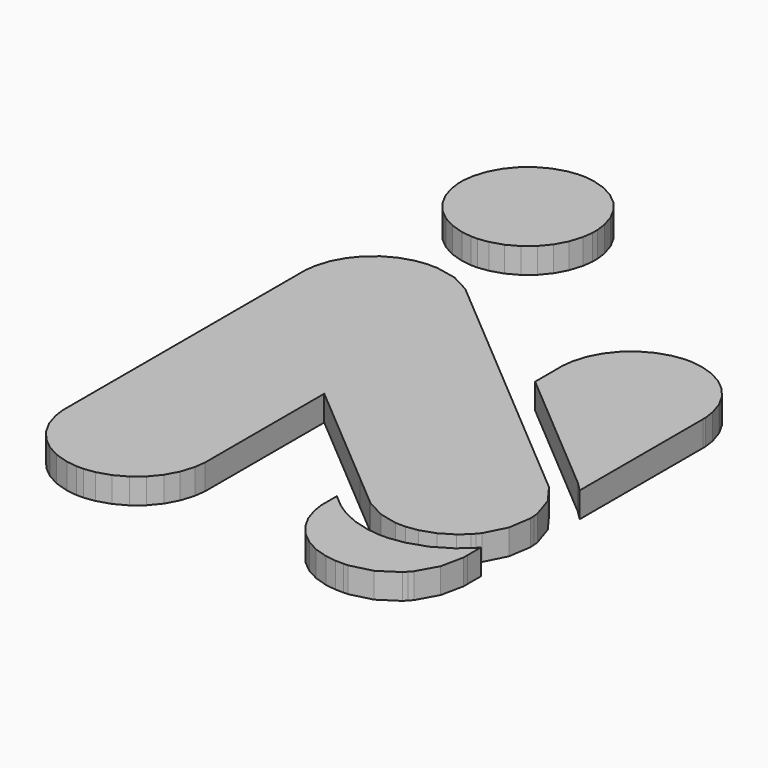
from build123d import *

# Parameters (mm, degrees)
F1_DEPTH = 0.15
F2_SCALE = 4


# Not quite as in the source:
# - ends of sketch curves that miss each other by under 0.0002 mm in the source are joined


with BuildPart() as f1:
    # F0 (on Top) → F1 (new body)
    with BuildSketch(Plane.XY):
        Polygon((-0.66371, 2.45638), (-0.68363, 2.45638), (-0.70359, 2.45638), (-0.76332, 2.44835), (-0.8376, 2.42524), (-0.90488, 2.38867), (-0.96346, 2.34027), (-1.01186, 2.28169), (-1.04843, 2.21441), (-1.07154, 2.14013), (-1.07957, 2.0804), (-1.07957, 2.06044), (-1.07957, 2.04052), (-1.07154, 1.9808), (-1.04843, 1.90652), (-1.01186, 1.8393), (-0.96346, 1.78065), (-0.90488, 1.73231), (-0.8376, 1.69574), (-0.76332, 1.67263), (-0.70359, 1.66455), (-0.68363, 1.66455), (-0.66371, 1.66455), (-0.60399, 1.67263), (-0.52971, 1.69574), (-0.46243, 1.73231), (-0.40384, 1.78065), (-0.35545, 1.8393), (-0.31893, 1.90652), (-0.29582, 1.9808), (-0.28774, 2.04052), (-0.28774, 2.06044), (-0.28774, 2.0804), (-0.29582, 2.14013), (-0.31893, 2.21441), (-0.35545, 2.28169), (-0.40384, 2.34027), (-0.46243, 2.38867), (-0.52971, 2.42524), (-0.60399, 2.44835), align=None)
    extrude(amount=F1_DEPTH)


with BuildPart() as f1b:
    # F0 (on Top) → F1, piece 2 (new body)
    with BuildSketch(Plane.XY):
        Polygon((-0.25009, -0.8451), (-0.25009, 0.01508), (0.41001, -0.54476), (0.57864, -0.68777), (0.59751, -0.70383), (0.70537, -0.76162), (0.81361, -0.78733), (0.84973, -0.78733), (0.87241, -0.78733), (0.94057, -0.7774), (1.02601, -0.74859), (1.10332, -0.70215), (1.15491, -0.65663), (1.16962, -0.63938), (1.18773, -0.61801), (1.24932, -0.49653), (1.2701, -0.36192), (1.26782, -0.33404), (1.26548, -0.3061), (1.22305, -0.17665), (1.14254, -0.06679), (1.12122, -0.04872), (0.31979, 0.63091), (-0.37688, 1.22178), (-0.39603, 1.23801), (-0.50518, 1.29606), (-0.62671, 1.32117), (-0.652, 1.32091), (-0.65352, 1.32085), (-0.65764, 1.32102), (-0.65861, 1.32108), (-0.66649, 1.32128), (-0.6694, 1.32128), (-0.69052, 1.32128), (-0.75384, 1.31277), (-0.8325, 1.28835), (-0.90368, 1.24967), (-0.96574, 1.19845), (-1.01702, 1.1364), (-1.0557, 1.06522), (-1.08017, 0.9866), (-1.08868, 0.92334), (-1.08868, 0.90223), (-1.08868, -0.8451), (-1.08868, -0.86616), (-1.08017, -0.92948), (-1.0557, -1.00809), (-1.01702, -1.07927), (-0.96574, -1.14133), (-0.90368, -1.19255), (-0.8325, -1.23123), (-0.75384, -1.25565), (-0.69052, -1.26422), (-0.6694, -1.26422), (-0.64836, -1.26422), (-0.58504, -1.25565), (-0.50638, -1.23123), (-0.43514, -1.19255), (-0.37309, -1.14133), (-0.32181, -1.07927), (-0.28313, -1.00809), (-0.25866, -0.92948), (-0.25009, -0.86616), align=None)
    extrude(amount=F1_DEPTH)


with BuildPart() as f1c:
    # F0 (on Top) → F1, piece 3 (new body)
    with BuildSketch(Plane.XY):
        Polygon((0.85348, 1.32128), (0.84996, 1.32128), (0.8288, 1.32112), (0.76543, 1.31201), (0.68687, 1.28678), (0.61596, 1.2474), (0.55428, 1.19558), (0.50361, 1.13302), (0.46557, 1.06147), (0.4418, 0.98258), (0.43389, 0.91916), (0.43411, 0.89806), (0.43416, 0.71609), (1.21107, 0.05719), (1.21665, 0.05246), (1.26819, 0.00135), (1.27291, -0.00413), (1.27265, 0.90658), (1.27243, 0.92746), (1.26337, 0.99002), (1.23847, 1.06776), (1.19946, 1.13819), (1.14814, 1.19959), (1.08618, 1.25033), (1.01526, 1.28863), (0.93714, 1.31288), (0.87437, 1.32128), align=None)
    extrude(amount=F1_DEPTH)


with BuildPart() as f1d:
    # F0 (on Top) → F1, piece 4 (new body)
    with BuildSketch(Plane.XY):
        Polygon((1.14407, -1.15072), (1.16229, -1.13102), (1.18041, -1.11133), (1.2453, -0.99469), (1.2734, -0.86035), (1.27314, -0.83181), (1.27308, -0.73199), (1.25355, -0.75467), (1.18508, -0.8144), (1.08276, -0.87538), (0.96975, -0.9132), (0.87975, -0.92622), (0.84973, -0.92622), (0.82522, -0.92622), (0.75182, -0.91748), (0.65753, -0.89198), (0.56908, -0.85048), (0.50746, -0.80952), (0.48879, -0.79373), (0.43454, -0.74773), (0.43459, -0.84034), (0.43476, -0.86117), (0.44382, -0.92367), (0.46878, -1.00147), (0.50778, -1.07188), (0.55911, -1.1333), (0.62107, -1.18403), (0.69197, -1.22233), (0.7701, -1.24659), (0.83282, -1.25505), (0.85376, -1.25505), (0.85673, -1.25505), (0.8658, -1.25505), (0.87562, -1.25505), (0.87893, -1.25505), (0.90643, -1.25477), (1.03458, -1.22223), align=None)
    extrude(amount=F1_DEPTH)


with BuildPart() as f1_1:
    # F2: moved
    add(f1.part.scale(F2_SCALE))


with BuildPart() as f1b_1:
    # F2: moved
    add(f1b.part.scale(F2_SCALE))


with BuildPart() as f1c_1:
    # F2: moved
    add(f1c.part.scale(F2_SCALE))


with BuildPart() as f1d_1:
    # F2: moved
    add(f1d.part.scale(F2_SCALE))


solid = Compound([f1_1.part, f1b_1.part, f1c_1.part, f1d_1.part])
